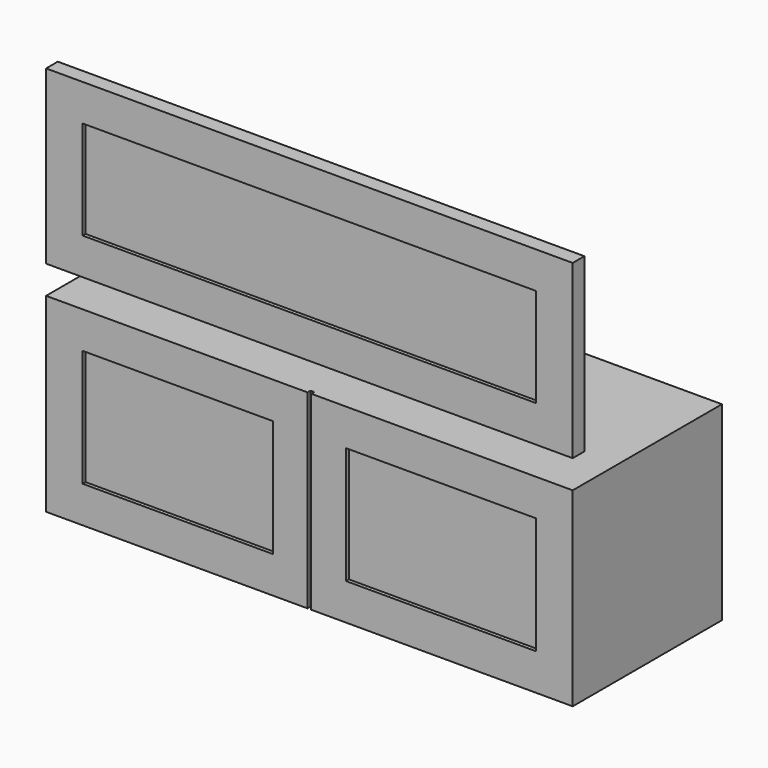
from build123d import *

# Parameters (mm, degrees)
F0_W     = 330.2
F0_H     = 203.2
F0_W_2   = 3.175
F0_H_2   = 330.2
F1_DEPTH = 323.85
F2_DEPTH = 6.35
F0_W_3   = 914.4
F0_H_3   = 298.45
F0_W_4   = 787.4
F0_H_4   = 171.45
F3_DEPTH = 25.4
F4_DEPTH = 6.35


# Not quite as in the source:
# - a feature names something its author has since deleted; it is built from what else it names


with BuildPart() as f1:
    # F0 (on Front) → F1 (new body)
    with BuildSketch(Plane.XZ):
        Polygon((-229.2927574873, 0), (224.7322425127, 0), (224.7322425127, 330.2), (100.9072425127, 330.2), (-229.2927574873, 330.2), align=None)
        with Locations((-0.6927574873, 165.1)):
            Rectangle(F0_W, F0_H, mode=Mode.SUBTRACT)
        Polygon((231.0822425127, 330.2), (231.0822425127, 0), (685.1072425127, 0), (685.1072425127, 330.2), (354.9072425127, 330.2), align=None)
        with Locations((456.5072425127, 165.1)):
            Rectangle(F0_W, F0_H, mode=Mode.SUBTRACT)
        with Locations((-0.6927574873, 165.1)):
            Rectangle(F0_W, F0_H)
        with Locations((456.5072425127, 165.1)):
            Rectangle(F0_W, F0_H)
        with Locations((226.3197425127, 165.1)):
            Rectangle(F0_W_2, F0_H_2)
        with Locations((229.4947425127, 165.1)):
            Rectangle(F0_W_2, F0_H_2)
    extrude(amount=-F1_DEPTH)

    # F0 (on Front) → F2 (cut)
    with BuildSketch(Plane.XZ):
        with Locations((226.3197425127, 165.1)):
            Rectangle(F0_W_2, F0_H_2)
        with Locations((229.4947425127, 165.1)):
            Rectangle(F0_W_2, F0_H_2)
        with Locations((-0.6927574873, 165.1)):
            Rectangle(F0_W, F0_H)
        with Locations((456.5072425127, 165.1)):
            Rectangle(F0_W, F0_H)
    extrude(amount=-F2_DEPTH, mode=Mode.SUBTRACT)


with BuildPart() as f3:
    # F0 (on Front) → F3 (new body)
    with BuildSketch(Plane.XZ):
        with Locations((227.9072425127, 528.5571549892)):
            Rectangle(F0_W_3, F0_H_3)
        with Locations((227.9072425127, 528.5571549892)):
            Rectangle(F0_W_4, F0_H_4, mode=Mode.SUBTRACT)
        with Locations((227.9072425127, 528.5571549892)):
            Rectangle(F0_W_4, F0_H_4)
    extrude(amount=-F3_DEPTH)

    # F0 (on Front) → F4 (cut)
    with BuildSketch(Plane.XZ):
        with Locations((227.9072425127, 528.5571549892)):
            Rectangle(F0_W_4, F0_H_4)
    extrude(amount=-F4_DEPTH, mode=Mode.SUBTRACT)


solid = Compound([f1.part, f3.part])
